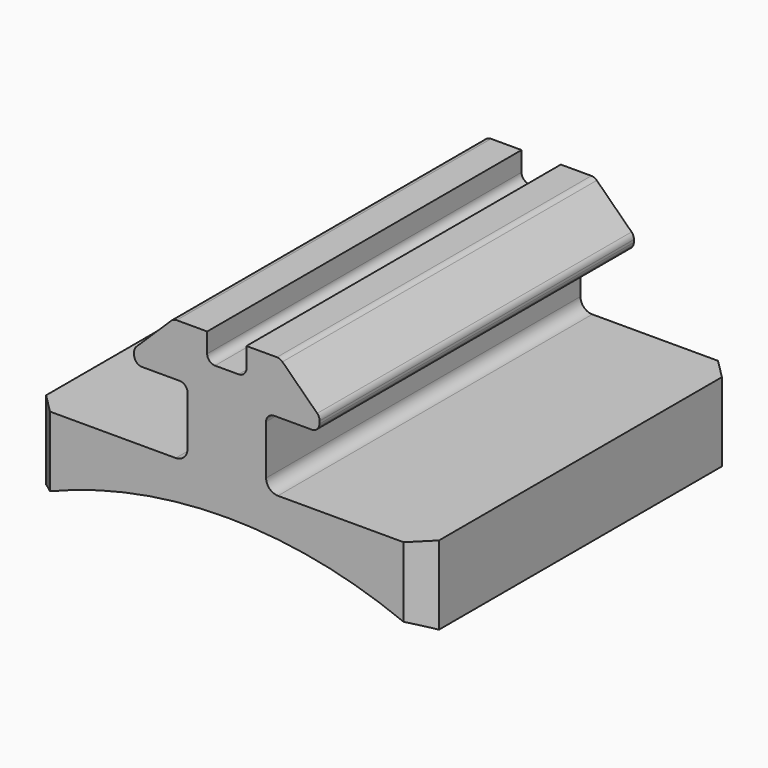
from build123d import *

# Parameters (mm, degrees)
F1_DEPTH = 10
F2_R     = 0.2
F3_R     = 0.3
F4_SIZE  = 0.5


# Not quite as in the source:
# - a feature names something its author has since deleted; it is built from what else it names


with BuildPart() as f1:
    # F0 (on Front) → F1 (new body)
    with BuildSketch(Plane.XZ):
        with BuildLine():
            Line((-5, 0.8663841993), (-5, -1.1336158007))
            ThreePointArc((-5, -1.1336158007), (-2.5588527336, -0.3183237919), (0, -0.0423279154))
            ThreePointArc((0, -0.0423279154), (2.5588527336, -0.3183237919), (5, -1.1336158007))
            Line((5, -1.1336158007), (5, 0.8663841993))
            Line((5, 0.8663841993), (1, 0.8663841993))
            Line((1, 0.8663841993), (1, 2.6280805469))
            Line((1, 2.6280805469), (2.3511576001, 2.6280805469))
            Line((2.3511576001, 2.6280805469), (2.363298554, 2.9764297366))
            Line((2.363298554, 2.9764297366), (1.357049332, 3.9621986704))
            Line((1.357049332, 3.9621986704), (0.5, 3.9621986704))
            Line((0.5, 3.9621986704), (0.5, 3.2621986704))
            Line((0.5, 3.2621986704), (0, 3.2621986704))
            Line((0, 3.2621986704), (-0.5, 3.2621986704))
            Line((-0.5, 3.2621986704), (-0.5, 3.9621986704))
            Line((-0.5, 3.9621986704), (-1.357049332, 3.9621986704))
            Line((-1.357049332, 3.9621986704), (-2.363298554, 2.9764297366))
            Line((-2.363298554, 2.9764297366), (-2.3511576001, 2.6280805469))
            Line((-2.3511576001, 2.6280805469), (-1, 2.6280805469))
            Line((-1, 2.6280805469), (-1, 0.8663841993))
            Line((-1, 0.8663841993), (-5, 0.8663841993))
        make_face()
    extrude(amount=F1_DEPTH)

    # F2
    f2_edges = [f1.edges().sort_by_distance(p)[0] for p in [
        (-0.5, -5, 3.262199),
        (0.5, -5, 3.262199),
        (2.351158, -5, 2.628081),
        (1, -5, 2.628081),
        (2.363299, -5, 2.97643),
        (1.357049, -5, 3.962199),
        (-1, -5, 2.628081),
        (-2.351158, -5, 2.628081),
        (-2.363299, -5, 2.97643),
        (-1.357049, -5, 3.962199),
    ]]
    fillet(f2_edges, radius=F2_R)

    # F3
    f3_edges = [f1.edges().sort_by_distance(p)[0] for p in [
        (-1, -5, 0.866384),
        (1, -5, 0.866384),
    ]]
    fillet(f3_edges, radius=F3_R)

    # F4
    f4_edges = [f1.edges().sort_by_distance(p)[0] for p in [
        (-5, -10, -0.133616),
        (5, -10, -0.133616),
        (5, 0, -0.133616),
        (-5, 0, -0.133616),
    ]]
    chamfer(f4_edges, length=F4_SIZE)


solid = f1.part
